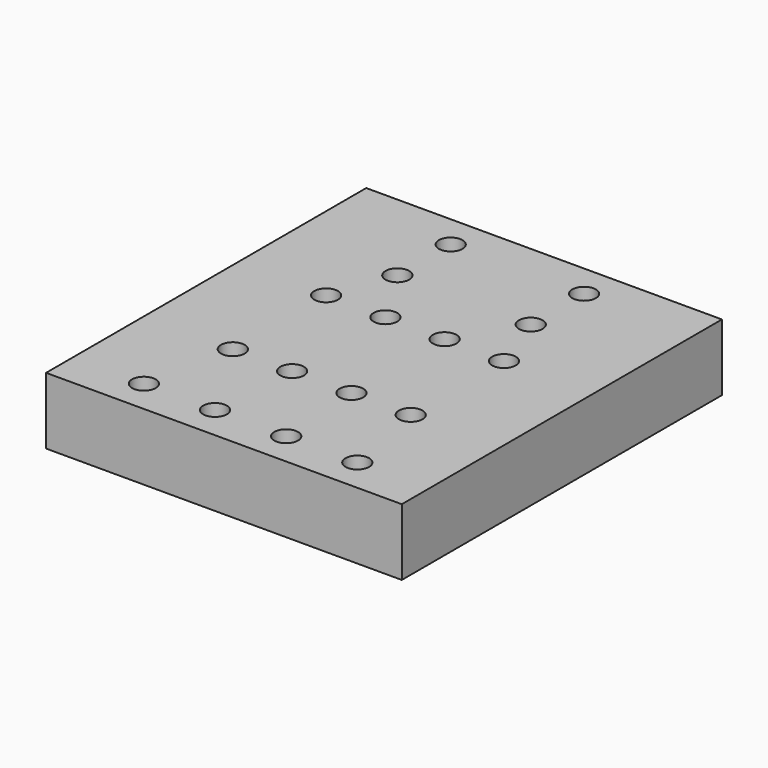
from build123d import *

# Parameters (mm, degrees)
F0_W     = 101.6
F0_H     = 114.3
F1_DEPTH = 19.05
F3_D     = 6.7564


# Not quite as in the source:
# - a feature names something its author has since deleted; it is built from what else it names


with BuildPart() as f1:
    # F0 (on Top) → F1 (new body)
    with BuildSketch(Plane.XY):
        Rectangle(F0_W, F0_H)
    extrude(amount=F1_DEPTH)

    # F3 (through all)
    with Locations(Plane.XY.offset(19.05)):
        with Locations((-30.48, -47.625), (-10.16, -47.625), (10.16, -47.625), (30.48, -47.625), (-19.05, 47.625), (-25.4, 11.0744), (-25.4, -22.225), (-8.4666666667, -22.225), (-8.4666666667, 11.0744), (8.4666666667, 11.0744), (8.4666666667, -22.225), (25.4, -22.225), (25.4, 11.0744), (19.05, 47.625), (-19.05, 28.575), (19.05, 28.575)):
            Hole(F3_D / 2)


solid = f1.part
